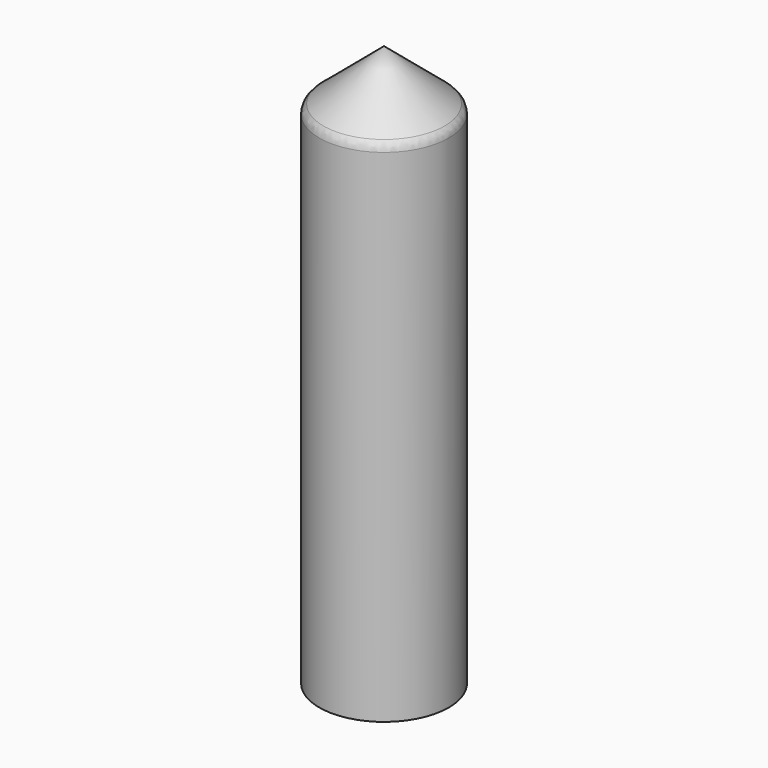
from build123d import *

# Parameters (mm, degrees)
F0_R     = 13.786
F0_R_2   = 11.5
F1_DEPTH = 107.95
F2_R     = 13.786
F2_R_2   = 11.5
F3_DEPTH = 31.75
F3_TAPER = 50
F4_T     = 2.54
F5_COUNT = 4
F6_R     = 2.54
F6_2_R   = 2.54
F6_3_R   = 2.54
F6_4_R   = 2.54


# Not quite as in the source:
# - a shell that OpenCascade refuses in one call is made with other operations: the cavity is built on its own and cut out
# - a feature names something its author has since deleted; it is built from what else it names


with BuildPart() as f1:
    # F0 (on Top) → F1 (new body)
    with BuildSketch(Plane.XY):
        Circle(F0_R)
        Circle(F0_R_2, mode=Mode.SUBTRACT)
    extrude(amount=F1_DEPTH)

    # F2 (on face) → F3 (join)
    with BuildSketch(Plane.XY.offset(107.95)):
        Circle(F2_R)
        Circle(F2_R_2, mode=Mode.SUBTRACT)
        Circle(F2_R_2)
    extrude(amount=F3_DEPTH, taper=F3_TAPER)

    # F4: shell of thickness 2.54, made by hand


with BuildPart() as f4_core1:
    # F4_t2: copy of F1
    add(f1.part)

    # the walls: a layer under each face that stays
    f4_faces = [f4_core1.faces().sort_by_distance(p)[0] for p in [
        (-13.786, 0, 53.975),
        (-9.1906666667, -9.1906666667, 0),
        (-6.893, 0, 113.7339137577),
        (-11.5, 0, 53.975),
    ]]
    thicken(f4_faces, amount=-F4_T, mode=Mode.SUBTRACT)


with BuildPart() as f1_1:
    add(f1.part)

    # what is left inside the walls is the cavity
    f4_cavity = [f4_core1.part.solids().sort_by_distance(p)[0] for p in [
        (-6.539981, 0, 110.68124),
    ]]
    add(f4_cavity, mode=Mode.SUBTRACT)


with BuildPart() as f5_1:
    # F5: instance of F1
    add(f1_1.part.rotate(Axis((0, 0, 0), (0, 0, 1)), 1 * 360 / F5_COUNT))

    # F6#2
    f6_2_edges = [f5_1.edges().sort_by_distance(p)[0] for p in [
        (0, -13.786, 107.95),
    ]]
    fillet(f6_2_edges, radius=F6_2_R)


with BuildPart() as f5_2:
    # F5: instance of F1
    add(f1_1.part.rotate(Axis((0, 0, 0), (0, 0, 1)), 2 * 360 / F5_COUNT))

    # F6#3
    f6_3_edges = [f5_2.edges().sort_by_distance(p)[0] for p in [
        (13.786, 0, 107.95),
    ]]
    fillet(f6_3_edges, radius=F6_3_R)


with BuildPart() as f5_3:
    # F5: instance of F1
    add(f1_1.part.rotate(Axis((0, 0, 0), (0, 0, 1)), 3 * 360 / F5_COUNT))

    # F6#4
    f6_4_edges = [f5_3.edges().sort_by_distance(p)[0] for p in [
        (0, 13.786, 107.95),
    ]]
    fillet(f6_4_edges, radius=F6_4_R)


with BuildPart() as f1_2:
    add(f1_1.part)

    # F6
    f6_edges = [f1_2.edges().sort_by_distance(p)[0] for p in [
        (-13.786, 0, 107.95),
        (6.893, 0, 113.733914),
    ]]
    fillet(f6_edges, radius=F6_R)


solid = f1_2.part
